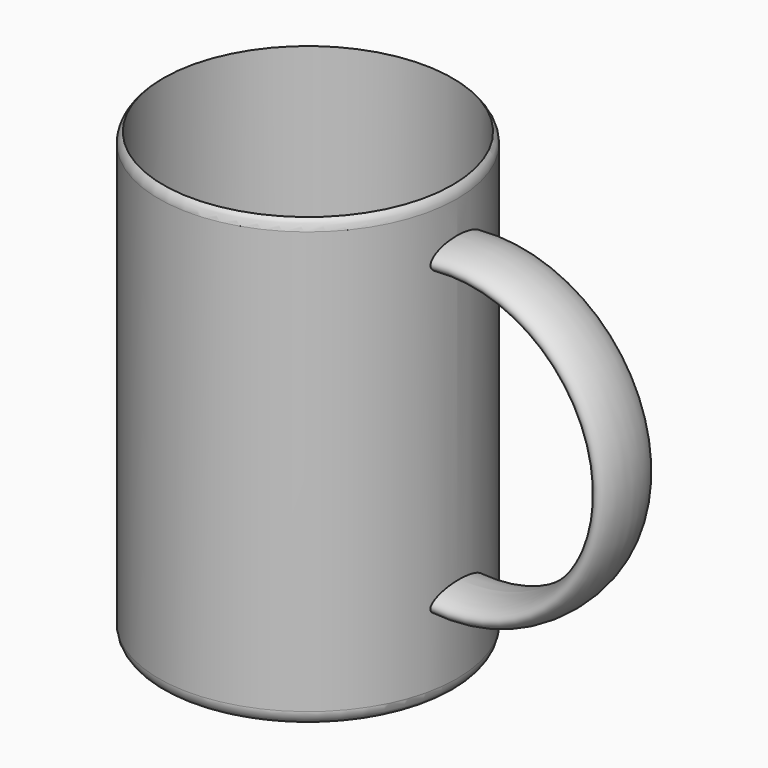
from build123d import *

# Parameters (mm, degrees)
F0_R     = 50.8
F0_R_2   = 49.2125
F1_DEPTH = 152.4
F2_DEPTH = 3.175
F7_R     = 5.08


# Not quite as in the source:
# - a fillet or chamfer that OpenCascade refuses, or shapes differently, is made with other operations: its cross-section is extruded or revolved along the edge and cut away or added


with BuildPart() as f1:
    # F0 (on Top) → F1 (new body)
    with BuildSketch(Plane.XY):
        with Locations((-50.7995303897, 0.2184311975)):
            Circle(F0_R)
        with Locations((-50.7995303897, 0.2184311975)):
            Circle(F0_R_2, mode=Mode.SUBTRACT)
    extrude(amount=F1_DEPTH)

    # F0 (on Top) → F2 (join)
    with BuildSketch(Plane.XY):
        with Locations((-50.7995303897, 0.2184311975)):
            Circle(F0_R_2)
    extrude(amount=F2_DEPTH)

    # F5: sweep along a path in F4
    with BuildLine(Plane.XZ) as f5_path:
        ThreePointArc((0, 31.0402940959), (56.0160848718, 82.0873966441), (0, 133.1344991922))
    # F3 (on Right) → F5 (sweep)
    with BuildSketch(Plane.YZ):
        with BuildLine():
            add(Edge.make_bspline(
                [(11.1326146871, 133.4060281515), (11.1326146871, 141.0279565911), (-5.5663073435, 137.2169923713), (-22.2652293742, 133.4060281515), (-5.5663073435, 129.5950639317), (11.1326146871, 125.7840997119), (11.1326146871, 133.4060281515)],
                knots=[0, 0, 0, 2.0943951024, 2.0943951024, 4.1887902048, 4.1887902048, 6.2831853072, 6.2831853072, 6.2831853072], degree=2, weights=[1, 0.5, 1, 0.5, 1, 0.5, 1]))
        make_face()
    sweep(path=f5_path.line)

    # F6: fillet of radius 5.08 on 1 edges, made by hand

    # F6_s1 → F6_t2 (revolve, cut)
    with BuildSketch(Plane.XZ.offset(-0.2184311975)):
        with BuildLine():
            ThreePointArc((0.0008696103, 148.7105678213), (-0.412881514, 150.7189630856), (-1.5867553659, 152.4002904513))
            Line((-1.5867553659, 152.4002904513), (-1.237381295, 152.7692627143))
            ThreePointArc((-1.237381295, 152.7692627143), (-0.7931428778, 152.9081365685), (0.0004696103, 152.9081365685))
            Line((0.0004696103, 152.9081365685), (0.5086061789, 152.4))
            ThreePointArc((0.5086061789, 152.4), (0.5086061789, 150.5552839107), (0.5090061789, 148.7105678213))
            Line((0.5090061789, 148.7105678213), (0.0008696103, 148.7105678213))
        make_face()
    revolve(axis=Axis((-50.7995303897, 0.2184311975, 152.4), (0, 0, 1)), mode=Mode.SUBTRACT)

    # F7
    f7_edges = [f1.edges().sort_by_distance(p)[0] for p in [
        (-101.59953, 0.218431, 0),
    ]]
    fillet(f7_edges, radius=F7_R)


solid = f1.part
